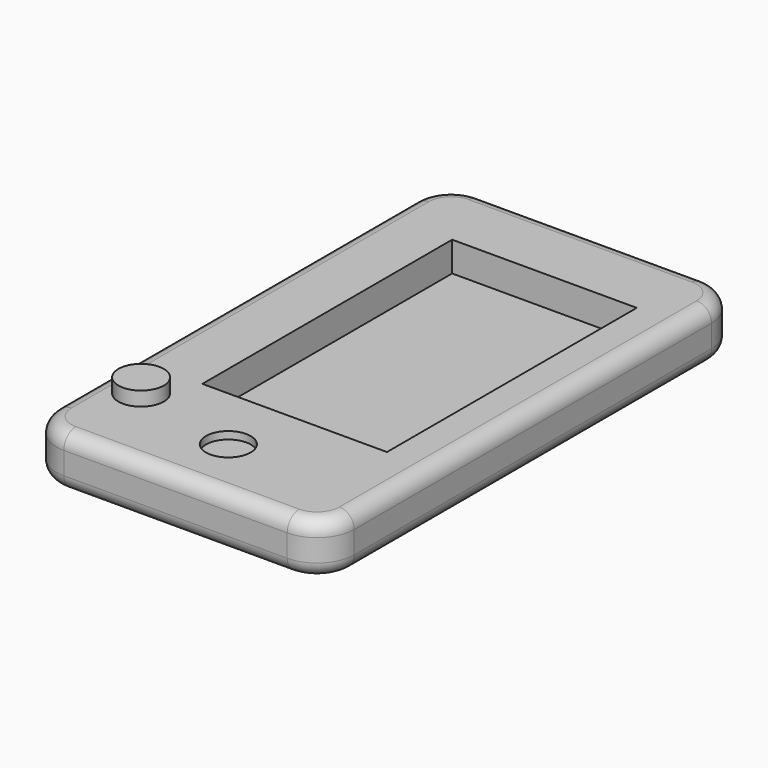
from build123d import *

# Parameters (mm, degrees)
F0_W         = 40
F0_H         = 70
F1_DEPTH     = 7
F2_R         = 5
F3_R         = 1.780942195
F4_DEPTH     = 3.7
F5_T1_DEPTH  = 60
F5_T3_DEPTH  = 30
F5_T6_ANGLE  = 90
F5_T8_ANGLE  = 90
F5_T10_ANGLE = 90
F5_T12_ANGLE = 90
F5_T14_ANGLE = 90
F5_T16_ANGLE = 90
F5_T18_ANGLE = 90
F5_T20_ANGLE = 90
F6_R         = 3
F7_DEPTH     = 1
F8_W         = 24.7989948839
F8_H         = 41.9472400099
F9_DEPTH     = 4
F10_R        = 3.0419567341
F11_DEPTH    = 1.9


# Not quite as in the source:
# - a fillet or chamfer that OpenCascade refuses, or shapes differently, is made with other operations: its cross-section is extruded or revolved along the edge and cut away or added


with BuildPart() as f1:
    # F0 (on Top) → F1 (new body)
    with BuildSketch(Plane.XY):
        with Locations((20, 35)):
            Rectangle(F0_W, F0_H)
    extrude(amount=F1_DEPTH)

    # F2
    f2_edges = [f1.edges().sort_by_distance(p)[0] for p in [
        (0, 0, 3.5),
        (40, 0, 3.5),
        (40, 70, 3.5),
        (0, 70, 3.5),
    ]]
    fillet(f2_edges, radius=F2_R)

    # F3 (on face) → F4 (cut)
    with BuildSketch(Plane(origin=(0, 70, 0), x_dir=(-1, 0, 0), z_dir=(0, 1, 0))):
        with Locations((-29.880721122, 3.5)):
            Circle(F3_R)
    extrude(amount=-F4_DEPTH, mode=Mode.SUBTRACT)

    # F5: fillet of radius 2 on 16 edges, made by hand

    # F5_s2 → F5_t1 (cut)
    with BuildSketch(Plane.XZ.offset(-65)):
        with BuildLine():
            ThreePointArc((38, 0), (39.4142135624, 0.5857864376), (40, 2))
            Line((40, 2), (40, 0))
            Line((40, 0), (38, 0))
        make_face()
        with BuildLine():
            ThreePointArc((38, 7), (39.4142135624, 6.4142135624), (40, 5))
            Line((40, 5), (40, 7))
            Line((40, 7), (38, 7))
        make_face()
        with BuildLine():
            ThreePointArc((0, 2), (0.5857864376, 0.5857864376), (2, 0))
            Line((2, 0), (0, 0))
            Line((0, 0), (0, 2))
        make_face()
        with BuildLine():
            ThreePointArc((0, 5), (0.5857864376, 6.4142135624), (2, 7))
            Line((2, 7), (0, 7))
            Line((0, 7), (0, 5))
        make_face()
    extrude(amount=F5_T1_DEPTH, mode=Mode.SUBTRACT)

    # F5_s4 → F5_t3 (cut)
    with BuildSketch(Plane.YZ.offset(5)):
        with BuildLine():
            ThreePointArc((68, 0), (69.4142135624, 0.5857864376), (70, 2))
            Line((70, 2), (70, 0))
            Line((70, 0), (68, 0))
        make_face()
        with BuildLine():
            ThreePointArc((2, 0), (0.5857864376, 0.5857864376), (0, 2))
            Line((0, 2), (0, 0))
            Line((0, 0), (2, 0))
        make_face()
        with BuildLine():
            ThreePointArc((68, 7), (69.4142135624, 6.4142135624), (70, 5))
            Line((70, 5), (70, 7))
            Line((70, 7), (68, 7))
        make_face()
        with BuildLine():
            ThreePointArc((2, 7), (0.5857864376, 6.4142135624), (0, 5))
            Line((0, 5), (0, 7))
            Line((0, 7), (2, 7))
        make_face()
    extrude(amount=F5_T3_DEPTH, mode=Mode.SUBTRACT)

    # F5_s5 → F5_t6 (revolve, cut)
    with BuildSketch(Plane.XZ.offset(-65)):
        with BuildLine():
            ThreePointArc((2, 0), (0.5857864376, 0.5857864376), (0, 2))
            Line((0, 2), (0, 0))
            Line((0, 0), (2, 0))
        make_face()
    revolve(axis=Axis((5, 65, 0), (0, 0, -1)), revolution_arc=F5_T6_ANGLE, mode=Mode.SUBTRACT)

    # F5_s7 → F5_t8 (revolve, cut)
    with BuildSketch(Plane.XZ.offset(-5)):
        with BuildLine():
            ThreePointArc((2, 0), (0.5857864376, 0.5857864376), (0, 2))
            Line((0, 2), (0, 0))
            Line((0, 0), (2, 0))
        make_face()
    revolve(axis=Axis((5, 5, 0), (0, 0, 1)), revolution_arc=F5_T8_ANGLE, mode=Mode.SUBTRACT)

    # F5_s9 → F5_t10 (revolve, cut)
    with BuildSketch(Plane.XZ.offset(-65)):
        with BuildLine():
            ThreePointArc((38, 0), (39.4142135624, 0.5857864376), (40, 2))
            Line((40, 2), (40, 0))
            Line((40, 0), (38, 0))
        make_face()
    revolve(axis=Axis((35, 65, 0), (0, 0, 1)), revolution_arc=F5_T10_ANGLE, mode=Mode.SUBTRACT)

    # F5_s11 → F5_t12 (revolve, cut)
    with BuildSketch(Plane.YZ.offset(35)):
        with BuildLine():
            ThreePointArc((2, 0), (0.5857864376, 0.5857864376), (0, 2))
            Line((0, 2), (0, 0))
            Line((0, 0), (2, 0))
        make_face()
    revolve(axis=Axis((35, 5, 0), (0, 0, 1)), revolution_arc=F5_T12_ANGLE, mode=Mode.SUBTRACT)

    # F5_s13 → F5_t14 (revolve, cut)
    with BuildSketch(Plane.XZ.offset(-65)):
        with BuildLine():
            ThreePointArc((0, 5), (0.5857864376, 6.4142135624), (2, 7))
            Line((2, 7), (0, 7))
            Line((0, 7), (0, 5))
        make_face()
    revolve(axis=Axis((5, 65, 7), (0, 0, -1)), revolution_arc=F5_T14_ANGLE, mode=Mode.SUBTRACT)

    # F5_s15 → F5_t16 (revolve, cut)
    with BuildSketch(Plane.XZ.offset(-5)):
        with BuildLine():
            ThreePointArc((0, 5), (0.5857864376, 6.4142135624), (2, 7))
            Line((2, 7), (0, 7))
            Line((0, 7), (0, 5))
        make_face()
    revolve(axis=Axis((5, 5, 7), (0, 0, 1)), revolution_arc=F5_T16_ANGLE, mode=Mode.SUBTRACT)

    # F5_s17 → F5_t18 (revolve, cut)
    with BuildSketch(Plane.XZ.offset(-65)):
        with BuildLine():
            ThreePointArc((38, 7), (39.4142135624, 6.4142135624), (40, 5))
            Line((40, 5), (40, 7))
            Line((40, 7), (38, 7))
        make_face()
    revolve(axis=Axis((35, 65, 7), (0, 0, 1)), revolution_arc=F5_T18_ANGLE, mode=Mode.SUBTRACT)

    # F5_s19 → F5_t20 (revolve, cut)
    with BuildSketch(Plane.YZ.offset(35)):
        with BuildLine():
            ThreePointArc((2, 7), (0.5857864376, 6.4142135624), (0, 5))
            Line((0, 5), (0, 7))
            Line((0, 7), (2, 7))
        make_face()
    revolve(axis=Axis((35, 5, 7), (0, 0, 1)), revolution_arc=F5_T20_ANGLE, mode=Mode.SUBTRACT)

    # F6 (on face) → F7 (cut)
    with BuildSketch(Plane.XY.offset(7)):
        with Locations((20, 8.8619329035)):
            Circle(F6_R)
    extrude(amount=-F7_DEPTH, mode=Mode.SUBTRACT)

    # F8 (on face) → F9 (cut)
    with BuildSketch(Plane.XY.offset(7)):
        with Locations((21.6991202906, 38.8473635539)):
            Rectangle(F8_W, F8_H)
    extrude(amount=-F9_DEPTH, mode=Mode.SUBTRACT)

    # F10 (on face) → F11 (join)
    with BuildSketch(Plane.XY.offset(7)):
        with Locations((5.6223799475, 12.1855456382)):
            Circle(F10_R)
    extrude(amount=F11_DEPTH)


solid = f1.part
